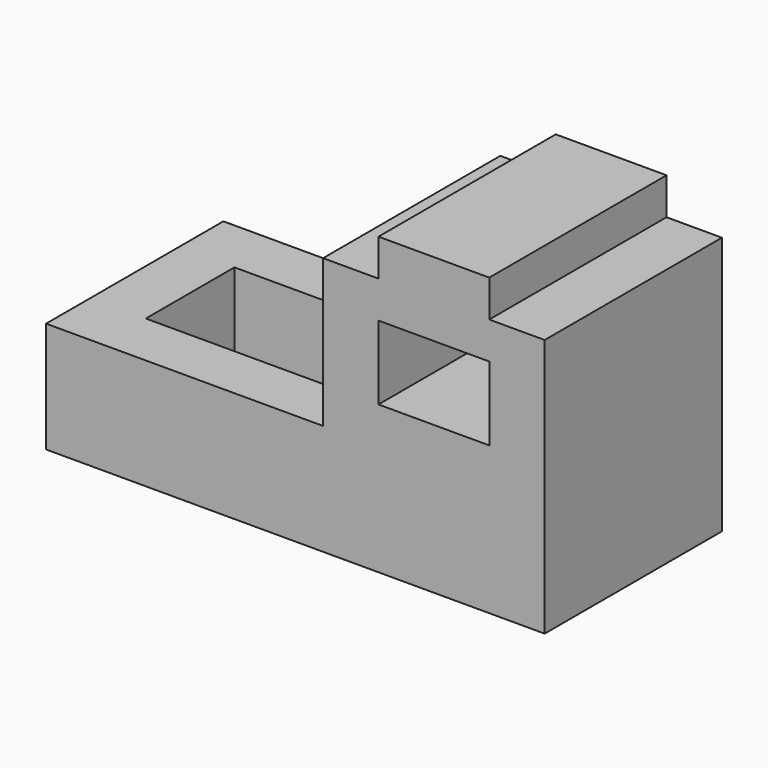
from build123d import *

# Parameters (mm, degrees)
F1_DEPTH = 1219.2
F2_W     = 609.6
F2_H     = 406.4
F3_DEPTH = 1219.2
F4_W     = 1219.2
F4_H     = 609.6
F5_DEPTH = 609.6


# Not quite as in the source:
# - a feature of the source that left no trace in its solid (it failed there, or was rolled back) is left out


with BuildPart() as f1:
    # F0 (on Front) → F1 (new body)
    with BuildSketch(Plane.XZ):
        Polygon((0, 609.6), (0, 0), (2743.2, 0), (2743.2, 1422.4), (2438.4, 1422.4), (2438.4, 1625.6), (1828.8, 1625.6), (1828.8, 1422.4), (1524, 1422.4), (1524, 609.6), align=None)
    extrude(amount=F1_DEPTH)

    # F2 (on face) → F3 (cut)
    with BuildSketch(Plane.XZ.offset(1219.2)):
        with Locations((2133.6, 1016)):
            Rectangle(F2_W, F2_H)
    extrude(amount=-F3_DEPTH, mode=Mode.SUBTRACT)

    # F4 (on face) → F5 (cut)
    with BuildSketch(Plane.XY.offset(609.6)):
        with Locations((914.4, -609.6)):
            Rectangle(F4_W, F4_H)
    extrude(amount=-F5_DEPTH, mode=Mode.SUBTRACT)


solid = f1.part
